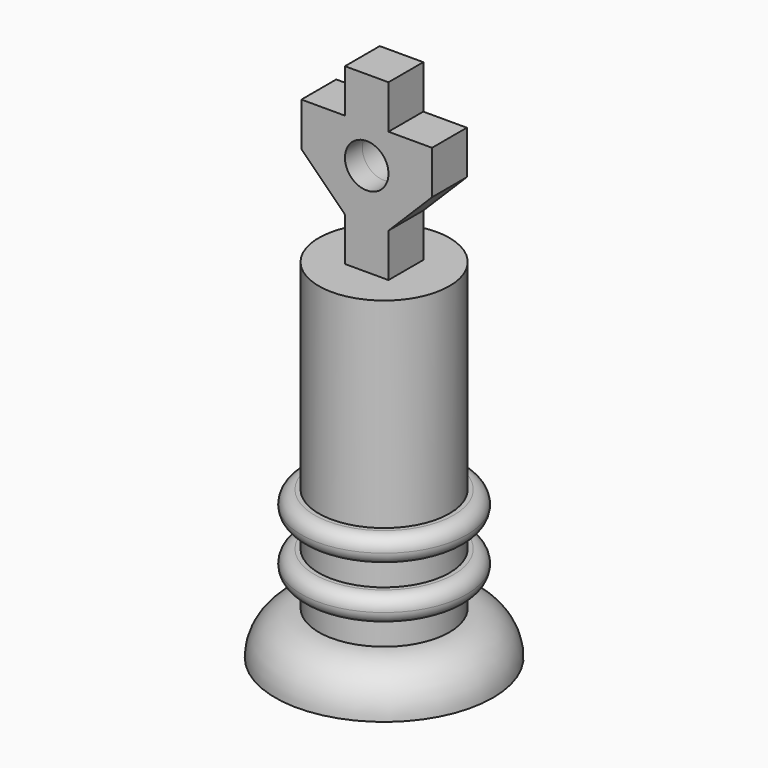
from build123d import *

# Parameters (mm, degrees)
F3_R           = 12.5
F3_R_2         = 9.5
F3_R_3         = 7.5
F4_DEPTH       = 5
F5_DEPTH       = 40
F6_START       = 8
F6_DEPTH       = 3
F7_START       = 14
F7_DEPTH       = 3
F8_R           = 1.49999
F9_R           = 1.49999
F10_R          = 4.99999
F14_R          = 2.5
F15_DEPTH      = 2.5
F15_DEPTH_BACK = 2.5
F16_SIZE       = 4.99999


# Not quite as in the source:
# - a fillet or chamfer is up to 0.001 mm smaller than in the source, because OpenCascade refuses the exact size


with BuildPart() as f4:
    # F3 (on Top) → F4 (new body)
    with BuildSketch(Plane.XY):
        Circle(F3_R)
        Circle(F3_R_2, mode=Mode.SUBTRACT)
        Circle(F3_R_2)
        Circle(F3_R_3, mode=Mode.SUBTRACT)
        Circle(F3_R_3)
    extrude(amount=F4_DEPTH)

    # F3 (on Top) → F5 (join)
    with BuildSketch(Plane.XY):
        Circle(F3_R_3)
    extrude(amount=F5_DEPTH)

    # F3 (on Top) → F6 (join)
    with BuildSketch(Plane.XY.offset(F6_START)):
        Circle(F3_R_2)
        Circle(F3_R_3, mode=Mode.SUBTRACT)
    extrude(amount=F6_DEPTH)

    # F3 (on Top) → F7 (join)
    with BuildSketch(Plane.XY.offset(F7_START)):
        Circle(F3_R_2)
        Circle(F3_R_3, mode=Mode.SUBTRACT)
    extrude(amount=F7_DEPTH)

    # F8 (radius 1.5 in the source; OpenCascade refuses exactly that, so slightly less here)
    f8_edges = [f4.edges().sort_by_distance(p)[0] for p in [
        (-9.5, 0, 8),
        (-9.5, 0, 11),
    ]]
    fillet(f8_edges, radius=F8_R)

    # F9 (radius 1.5 in the source; OpenCascade refuses exactly that, so slightly less here)
    f9_edges = [f4.edges().sort_by_distance(p)[0] for p in [
        (-9.5, 0, 14),
        (-9.5, 0, 17),
    ]]
    fillet(f9_edges, radius=F9_R)

    # F10 (radius 5 in the source; OpenCascade refuses exactly that, so slightly less here)
    f10_edges = [f4.edges().sort_by_distance(p)[0] for p in [
        (-12.5, 0, 5),
    ]]
    fillet(f10_edges, radius=F10_R)

    # F14 (on Front) → F15 (join, two sides)
    with BuildSketch(Plane.XZ) as f15_sk:
        Polygon((-2.5, 50), (-2.5, 40), (2.5, 40), (2.5, 50), (7.5, 50), (7.5, 55), (2.5, 55), (2.5, 60), (-2.5, 60), (-2.5, 55), (-7.5, 55), (-7.5, 50), align=None)
        with Locations((0, 50.75)):
            Circle(F14_R, mode=Mode.SUBTRACT)
    extrude(amount=F15_DEPTH)
    extrude(f15_sk.sketch, amount=-F15_DEPTH_BACK)

    # F16 (size 5 in the source; OpenCascade refuses exactly that, so slightly less here)
    f16_edges = [f4.edges().sort_by_distance(p)[0] for p in [
        (-2.5, 0, 50),
        (2.5, 0, 50),
    ]]
    chamfer(f16_edges, length=F16_SIZE)


solid = f4.part
